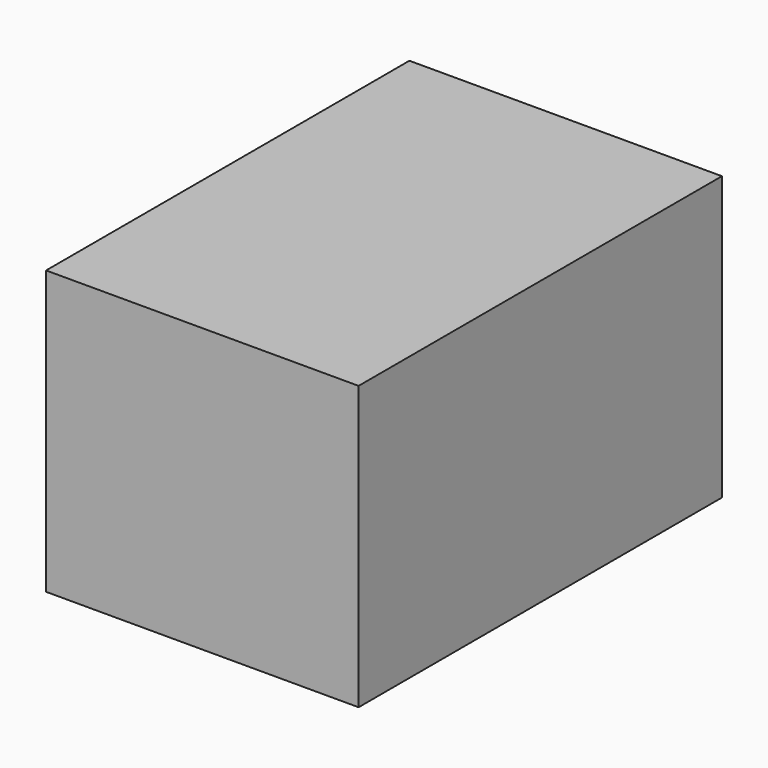
from build123d import *

# Parameters (mm, degrees)
F0_W          = 130.5738128722
F0_H          = 118.2156167924
F1_DEPTH      = 85.344
F1_DEPTH_BACK = 104.394


# Not quite as in the source:
# - a feature of the source that left no trace in its solid (it failed there, or was rolled back) is left out


with BuildPart() as f1:
    # F0 (on Front) → F1 (new body, two sides)
    with BuildSketch(Plane.XZ) as f1_sk:
        with Locations((8.1346090883, 0.3699008375)):
            Rectangle(F0_W, F0_H)
    extrude(amount=F1_DEPTH)
    extrude(f1_sk.sketch, amount=-F1_DEPTH_BACK)


solid = f1.part
